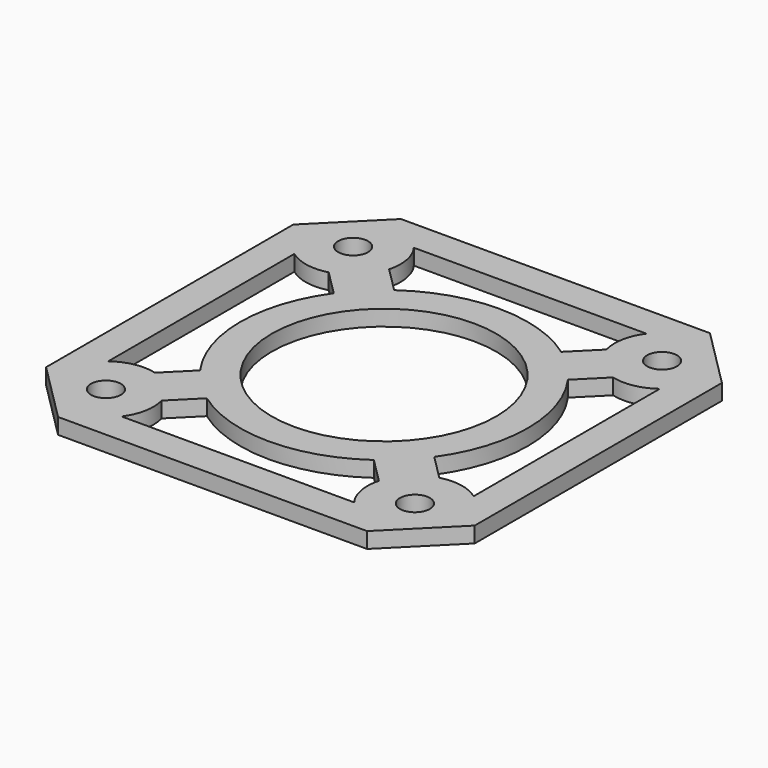
from build123d import *

# Parameters (mm, degrees)
F0_W            = 43.0059846
F0_H            = 43.0059846
F0_R            = 1.5
F0_R_2          = 11.2530001
F1_DEPTH        = 1.58115
F2_SIZE         = 6.0030106
F4_DEPTH        = 1.58115
F4_COPIES_COUNT = 4


# Not quite as in the source:
# - a pattern or mirror of a feature is missing from the dataset's text; its kind, count and spacing are read off the source's solid


with BuildPart() as f1:
    # F0 (on Top) → F1 (new body)
    with BuildSketch(Plane.XY):
        with Locations((21.5029923, 21.5029923)):
            Rectangle(F0_W, F0_H)
        with Locations((6.0029979, 6.0029979)):
            Circle(F0_R, mode=Mode.SUBTRACT)
        with Locations((21.5029923, 21.5029923)):
            Circle(F0_R_2, mode=Mode.SUBTRACT)
        with Locations((37.0029867, 6.0029979)):
            Circle(F0_R, mode=Mode.SUBTRACT)
        with Locations((6.0029979, 37.0029867)):
            Circle(F0_R, mode=Mode.SUBTRACT)
        with Locations((37.0029867, 37.0029867)):
            Circle(F0_R, mode=Mode.SUBTRACT)
    extrude(amount=F1_DEPTH)

    # F2
    f2_edges = [f1.edges().sort_by_distance(p)[0] for p in [
        (0, 0, 0.790575),
        (0, 43.005985, 0.790575),
        (43.005985, 0, 0.790575),
        (43.005985, 43.005985, 0.790575),
    ]]
    chamfer(f2_edges, length=F2_SIZE)

    # F3 (on face) → F4 (cut, through all)
    with BuildSketch(Plane.XY.offset(1.58115)):
        with BuildLine():
            ThreePointArc((7.2356236023, 32.4027649523), (5.1176370603, 32.3235056996), (3.175, 33.171037571))
            Line((3.175, 33.171037571), (3.175, 9.834947029))
            ThreePointArc((3.175, 9.834947029), (5.1176370603, 10.6824789004), (7.2356236023, 10.6032196477))
            Line((7.2356236023, 10.6032196477), (9.7569670059, 13.1245630513))
            ThreePointArc((9.7569670059, 13.1245630513), (7.0749922, 21.5029923), (9.7569670059, 29.8814215487))
            Line((9.7569670059, 29.8814215487), (7.2356236023, 32.4027649523))
        make_face()
    f4 = extrude(amount=-F4_DEPTH, mode=Mode.SUBTRACT)

    # F4_copies: F4 ×4 about axis
    f4_copies_axis = Axis((21.502992, 21.502992, 0), (0, 0, 1))
    for i in range(1, F4_COPIES_COUNT):
        add(f4.rotate(f4_copies_axis, i * 360 / F4_COPIES_COUNT), mode=Mode.SUBTRACT)


solid = f1.part
